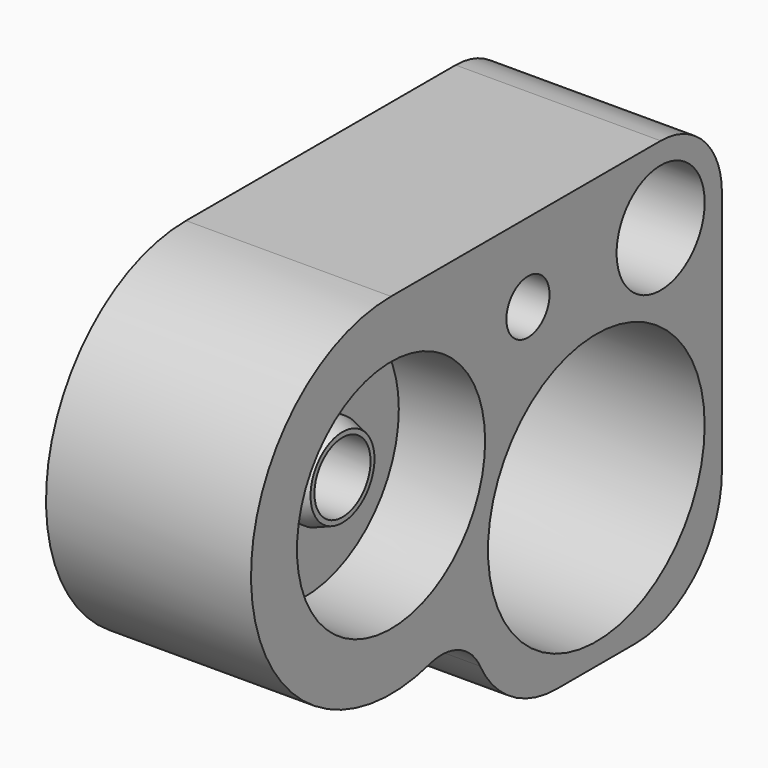
from build123d import *

# Parameters (mm, degrees)
F0_R          = 12.55
F0_R_2        = 10.9
F0_R_3        = 3.25
F0_R_4        = 5.1
F0_R_5        = 2.5
F1_DEPTH      = 9
F2_DEPTH      = 10
F3_R          = 10
F4_R          = 5
F11_DEPTH     = 2.9
F10_R         = 3.25
F13_T4_ANGLE  = 230.6618088311
F13_S5_R      = 3.25
F13_T6_DEPTH  = 6
F13_T10_ANGLE = 171.9012593912
F13_S11_R     = 3.25
F13_T12_DEPTH = 5


# Not quite as in the source:
# - a fillet or chamfer that OpenCascade refuses, or shapes differently, is made with other operations: its cross-section is extruded or revolved along the edge and cut away or added


with BuildPart() as f1:
    # F0 (on Right) → F1 (new body)
    with BuildSketch(Plane.YZ):
        with BuildLine():
            Line((7.45, 25.2829590551), (-23.7829060836, 25.2829590551))
            ThreePointArc((-23.7829060836, 25.2829590551), (-39.2686382031, 4.2232189691), (-14.55, -4.280278967))
            Line((-14.55, -4.280278967), (-14.55, -14.55))
            Line((-14.55, -14.55), (14.55, -14.55))
            Line((14.55, -14.55), (14.55, 18.1829590551))
            ThreePointArc((14.55, 18.1829590551), (12.4704581464, 23.2034172015), (7.45, 25.2829590551))
        make_face()
        Circle(F0_R, mode=Mode.SUBTRACT)
        with Locations((-23.7829060836, 9.059573843)):
            Circle(F0_R_2, mode=Mode.SUBTRACT)
        with Locations((-7.9205860656, 17.9829590551)):
            Circle(F0_R_3, mode=Mode.SUBTRACT)
        with Locations((7.45, 18.1829590551)):
            Circle(F0_R_4, mode=Mode.SUBTRACT)
        with Locations((-7.9205860656, 17.9829590551)):
            Circle(F0_R_3)
        with Locations((-7.9205860656, 17.9829590551)):
            Circle(F0_R_5, mode=Mode.SUBTRACT)
    extrude(amount=F1_DEPTH)

    # F0 (on Right) → F2 (join)
    with BuildSketch(Plane.YZ):
        with BuildLine():
            Line((7.45, 25.2829590551), (-23.7829060836, 25.2829590551))
            ThreePointArc((-23.7829060836, 25.2829590551), (-39.2686382031, 4.2232189691), (-14.55, -4.280278967))
            Line((-14.55, -4.280278967), (-14.55, -14.55))
            Line((-14.55, -14.55), (14.55, -14.55))
            Line((14.55, -14.55), (14.55, 18.1829590551))
            ThreePointArc((14.55, 18.1829590551), (12.4704581464, 23.2034172015), (7.45, 25.2829590551))
        make_face()
        Circle(F0_R, mode=Mode.SUBTRACT)
        with Locations((-23.7829060836, 9.059573843)):
            Circle(F0_R_2, mode=Mode.SUBTRACT)
        with Locations((-7.9205860656, 17.9829590551)):
            Circle(F0_R_3, mode=Mode.SUBTRACT)
        with Locations((7.45, 18.1829590551)):
            Circle(F0_R_4, mode=Mode.SUBTRACT)
        with Locations((-23.7829060836, 9.059573843)):
            Circle(F0_R_2)
    extrude(amount=-F2_DEPTH)

    # F3
    f3_edges = [f1.edges().sort_by_distance(p)[0] for p in [
        (-0.5, -23.782906, 25.282959),
        (-0.5, 14.55, 18.182959),
        (-0.5, 7.45, 25.282959),
        (-0.5, -14.55, -14.55),
        (-0.5, 14.55, -14.55),
    ]]
    fillet(f3_edges, radius=F3_R)

    # F4
    f4_edges = [f1.edges().sort_by_distance(p)[0] for p in [
        (-0.5, -14.55, -4.280279),
    ]]
    fillet(f4_edges, radius=F4_R)

    # F7 (on plane+point) → F8 (revolve)
    with BuildSketch(Plane.XY.offset(9.059573843)):
        Polygon((1, -12.7829060836), (0, -12.7829060836), (0, -20.5329060836), (4.5, -20.5329060836), (4.5, -20.078861435), (3, -19.5329060836), (1, -19.5329060836), align=None)
    revolve(axis=Axis((4.5, -23.7829060836, 9.059573843), (1, 0, 0)))

    # F0 (on Right) → F11 (join)
    with BuildSketch(Plane.YZ):
        with Locations((-7.9205860656, 17.9829590551)):
            Circle(F0_R_3)
        with Locations((-7.9205860656, 17.9829590551)):
            Circle(F0_R_5, mode=Mode.SUBTRACT)
    extrude(amount=-F11_DEPTH)

    # F12: sweep along a path in F9
    with BuildLine(Plane(origin=(0, -9.5885144747, 17.044662029), x_dir=(1, 0, 0), z_dir=(0, 0.4902958908, -0.8715560449))) as f12_path:
        ThreePointArc((0, 16.2862637363), (-4.2426406871, 14.5289044234), (-6, 10.2862637363))
        Line((-6, 10.2862637363), (-6, -1.9137362637))
    # F10 (on face) → F12 (sweep, cut)
    with BuildSketch(Plane.YZ):
        with Locations((-23.7829060836, 9.059573843)):
            Circle(F10_R)
    sweep(path=f12_path.line, mode=Mode.SUBTRACT)

    # F13: chamfer of 0.75 on 1 edges, made by hand


with BuildPart() as f13_tool2:
    # F13_s3 → F13_t4 (revolve)
    with BuildSketch(Plane.XY.offset(17.9829590551)):
        Polygon((-2.9, -4.6705860656), (-2.15, -5.4205860656), (-2.9, -5.4205860656), align=None)
    revolve(axis=Axis((-2.9, -7.9205860656, 17.9829590551), (1, 0, 0)), revolution_arc=F13_T4_ANGLE)

    # F13_s5 → F13_t6 (intersect, symmetric)
    with BuildSketch(Plane.YZ.offset(-2.5)):
        with Locations((-7.9205860656, 17.9829590551)):
            Circle(F13_S5_R)
    extrude(amount=F13_T6_DEPTH, both=True, mode=Mode.INTERSECT)


with BuildPart() as f1_1:
    add(f1.part)

    # F13_t1: cut F13_tool2
    add(f13_tool2.part, mode=Mode.SUBTRACT)


with BuildPart() as f13_tool8:
    # F13_s9 → F13_t10 (revolve)
    with BuildSketch(Plane(origin=(0, -2.6653633076, 18.7307701592), x_dir=(1, 0, 0), z_dir=(0, -0.1408794707, 0.9900267546))):
        Polygon((-2.9, -8.558162364), (-2.15, -7.808162364), (-2.9, -7.808162364), align=None)
    revolve(axis=Axis((-2.9, -7.9205860656, 17.9829590551), (1, 0, 0)), revolution_arc=F13_T10_ANGLE)

    # F13_s11 → F13_t12 (intersect, symmetric)
    with BuildSketch(Plane.YZ.offset(-2.5)):
        with Locations((-7.9205860656, 17.9829590551)):
            Circle(F13_S11_R)
    extrude(amount=F13_T12_DEPTH, both=True, mode=Mode.INTERSECT)


with BuildPart() as f1_2:
    add(f1_1.part)

    # F13_t7: cut F13_tool8
    add(f13_tool8.part, mode=Mode.SUBTRACT)


solid = f1_2.part
